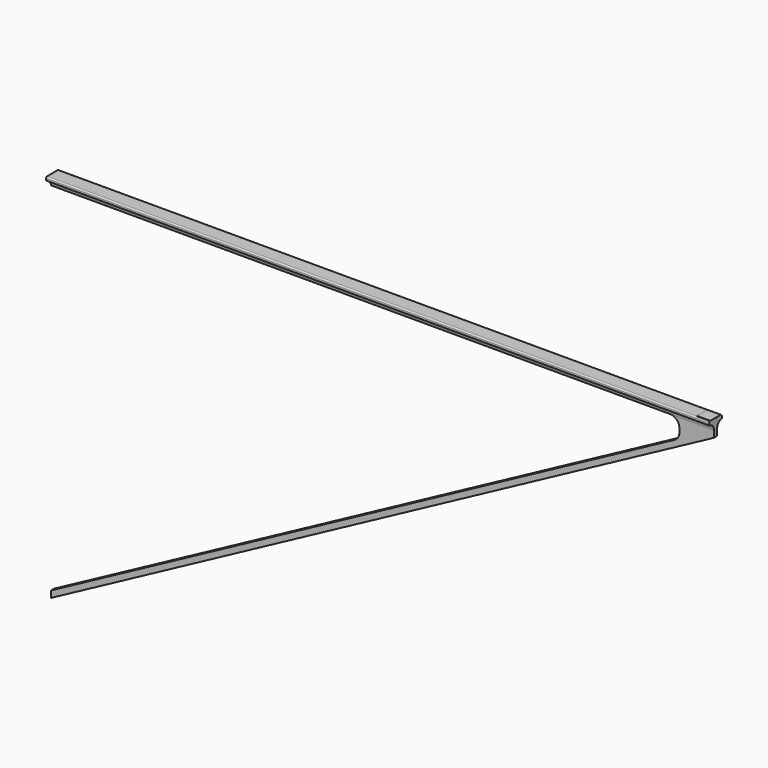
from build123d import *

# Parameters (mm, degrees)
F1_DEPTH      = 502
F3_DEPTH      = 406
F4_DEPTH      = 143
F5_W          = 26.22529459
F5_H          = 3
F6_DEPTH      = 14.25
F6_DEPTH_BACK = 0.8
F8_DEPTH      = 25
F10_DEPTH     = 0.27
F11_R         = 7
F12_R         = 7
F13_T1_DEPTH  = 502
F14_T1_DEPTH  = 502
F15_T1_DEPTH  = 507
F15_T6_DEPTH  = 507
F15_T12_DEPTH = 507
F15_T18_DEPTH = 507
F15_T25_DEPTH = 507
F15_T31_DEPTH = 507


# Not quite as in the source:
# - a fillet or chamfer that OpenCascade refuses, or shapes differently, is made with other operations: its cross-section is extruded or revolved along the edge and cut away or added
# - a feature names something its author has since deleted; it is built from what else it names


with BuildPart() as f1:
    # F0 (on Right) → F1 (new body)
    with BuildSketch(Plane.YZ):
        Polygon((6, 24.6420782059), (-6, 24.6420782059), (-6, 22.1420782059), (-1.5, 22.1420782059), (-1.5, -257.8579217941), (1.5, -257.8579217941), (1.5, 22.1420782059), (6, 22.1420782059), align=None)
    extrude(amount=F1_DEPTH)

    # F2 (on face) → F3 (cut)
    with BuildSketch(Plane.XZ.offset(1.5)):
        Polygon((0, -252.8579217941), (502, 17.1420782059), (0, 17.1420782059), align=None)
    extrude(amount=-F3_DEPTH, mode=Mode.SUBTRACT)

    # F2 (on face) → F4 (cut)
    with BuildSketch(Plane.XZ.offset(1.5)):
        Polygon((502, -257.8579217941), (502, 12.1420782059), (0, -257.8579217941), align=None)
    extrude(amount=-F4_DEPTH, mode=Mode.SUBTRACT)

    # F5 (on face) → F6 (join, two sides)
    with BuildSketch(Plane(origin=(0, 0, 17.1420782059), x_dir=(1, 0, 0), z_dir=(0, 0, -1))) as f6_sk:
        with Locations((488.887352705, 0)):
            Rectangle(F5_W, F5_H)
    extrude(amount=F6_DEPTH)
    extrude(f6_sk.sketch, amount=-F6_DEPTH_BACK)

    # F7 (on face) → F8 (cut)
    with BuildSketch(Plane(origin=(0, 1.5, 0), x_dir=(-1, 0, 0), z_dir=(0, 1, 0))):
        Polygon((-484.8018518519, 2.8920782059), (-502, 12.143202126), (-502, 2.8920782059), align=None)
    extrude(amount=-F8_DEPTH, mode=Mode.SUBTRACT)

    # F9 (on face) → F10 (join)
    with BuildSketch(Plane.XY.offset(24.6420782059)):
        Polygon((501.9800190187, -5.0222751118), (501.9800190187, 4.9777248882), (497.843503952, 4.9777248882), (491.9800190187, 4.9777248882), (491.9800190187, -5.0222751118), (496.5066611767, -5.0222751118), align=None)
    extrude(amount=F10_DEPTH)

    # F11
    f11_edges = [f1.edges().sort_by_distance(p)[0] for p in [
        (475.774705, 0, 17.142078),
    ]]
    fillet(f11_edges, radius=F11_R)

    # F12
    f12_edges = [f1.edges().sort_by_distance(p)[0] for p in [
        (475.774705, 0, 3.03684),
    ]]
    fillet(f12_edges, radius=F12_R)

    # F13: fillet of radius 5 on 1 edges, made by hand

    # F13_s2 → F13_t1 (join)
    with BuildSketch(Plane.YZ):
        with BuildLine():
            ThreePointArc((1.5, 17.1671410204), (2.7919007565, 20.5212429867), (6, 22.1420782059))
            Line((6, 22.1420782059), (1.5, 22.1420782059))
            Line((1.5, 22.1420782059), (1.5, 17.1671410204))
        make_face()
    extrude(amount=F13_T1_DEPTH)

    # F14: fillet of radius 5 on 1 edges, made by hand

    # F14_s2 → F14_t1 (join)
    with BuildSketch(Plane.YZ):
        with BuildLine():
            ThreePointArc((-1.5, 17.1671410204), (-2.7919007565, 20.5212429867), (-6, 22.1420782059))
            Line((-6, 22.1420782059), (-1.5, 22.1420782059))
            Line((-1.5, 22.1420782059), (-1.5, 17.1671410204))
        make_face()
    extrude(amount=F14_T1_DEPTH)

    # F15: fillet of radius 1 on 2 edges, made by hand

    # F15_s2 → F15_t1 (cut)
    with BuildSketch(Plane.YZ.offset(-2.5)):
        with BuildLine():
            ThreePointArc((6, 23.6420782059), (5.7071067812, 24.3491849871), (5, 24.6420782059))
            Line((5, 24.6420782059), (6, 24.6420782059))
            Line((6, 24.6420782059), (6, 23.6420782059))
        make_face()
    extrude(amount=F15_T1_DEPTH, mode=Mode.SUBTRACT)


with BuildPart() as f15_tool4:
    # F15_s5 → F15_t6 (new body)
    with BuildSketch(Plane.YZ.offset(-2.5)):
        with BuildLine():
            ThreePointArc((-5, 24.6420782059), (-5.7071067812, 24.3491849871), (-6, 23.6420782059))
            Line((-6, 23.6420782059), (-6, 24.6420782059))
            Line((-6, 24.6420782059), (-5, 24.6420782059))
        make_face()
    extrude(amount=F15_T6_DEPTH)

    split(bisect_by=Plane.YZ.offset(491.9800190187), keep=Keep.BOTTOM)

    split(bisect_by=Plane.XZ.offset(5.0222751118), keep=Keep.BOTTOM)


with BuildPart() as f1_1:
    add(f1.part)

    # F15_t3: cut F15_tool4
    add(f15_tool4.part, mode=Mode.SUBTRACT)


with BuildPart() as f15_tool10:
    # F15_s11 → F15_t12 (new body)
    with BuildSketch(Plane.YZ.offset(-2.5)):
        with BuildLine():
            ThreePointArc((-5, 24.6420782059), (-5.7071067812, 24.3491849871), (-6, 23.6420782059))
            Line((-6, 23.6420782059), (-6, 24.6420782059))
            Line((-6, 24.6420782059), (-5, 24.6420782059))
        make_face()
    extrude(amount=F15_T12_DEPTH)

    split(bisect_by=Plane.YZ.offset(491.9800190187), keep=Keep.BOTTOM)

    split(bisect_by=Plane.XZ.offset(5.0222751118), keep=Keep.TOP)


with BuildPart() as f1_2:
    add(f1_1.part)

    # F15_t9: cut F15_tool10
    add(f15_tool10.part, mode=Mode.SUBTRACT)


with BuildPart() as f15_tool16:
    # F15_s17 → F15_t18 (new body)
    with BuildSketch(Plane.YZ.offset(-2.5)):
        with BuildLine():
            ThreePointArc((-5, 24.6420782059), (-5.7071067812, 24.3491849871), (-6, 23.6420782059))
            Line((-6, 23.6420782059), (-6, 24.6420782059))
            Line((-6, 24.6420782059), (-5, 24.6420782059))
        make_face()
    extrude(amount=F15_T18_DEPTH)

    split(bisect_by=Plane.YZ.offset(491.9800190187), keep=Keep.TOP)

    split(bisect_by=Plane.YZ.offset(501.9800190187), keep=Keep.BOTTOM)

    split(bisect_by=Plane.XZ.offset(5.0222751118), keep=Keep.TOP)


with BuildPart() as f1_3:
    add(f1_2.part)

    # F15_t15: cut F15_tool16
    add(f15_tool16.part, mode=Mode.SUBTRACT)


with BuildPart() as f15_tool23:
    # F15_s24 → F15_t25 (new body)
    with BuildSketch(Plane.YZ.offset(-2.5)):
        with BuildLine():
            ThreePointArc((-5, 24.6420782059), (-5.7071067812, 24.3491849871), (-6, 23.6420782059))
            Line((-6, 23.6420782059), (-6, 24.6420782059))
            Line((-6, 24.6420782059), (-5, 24.6420782059))
        make_face()
    extrude(amount=F15_T25_DEPTH)

    split(bisect_by=Plane.YZ.offset(501.9800190187), keep=Keep.TOP)

    split(bisect_by=Plane.XZ.offset(5.0222751118), keep=Keep.BOTTOM)


with BuildPart() as f1_4:
    add(f1_3.part)

    # F15_t22: cut F15_tool23
    add(f15_tool23.part, mode=Mode.SUBTRACT)


with BuildPart() as f15_tool29:
    # F15_s30 → F15_t31 (new body)
    with BuildSketch(Plane.YZ.offset(-2.5)):
        with BuildLine():
            ThreePointArc((-5, 24.6420782059), (-5.7071067812, 24.3491849871), (-6, 23.6420782059))
            Line((-6, 23.6420782059), (-6, 24.6420782059))
            Line((-6, 24.6420782059), (-5, 24.6420782059))
        make_face()
    extrude(amount=F15_T31_DEPTH)

    split(bisect_by=Plane.YZ.offset(501.9800190187), keep=Keep.TOP)

    split(bisect_by=Plane.XZ.offset(5.0222751118), keep=Keep.TOP)


with BuildPart() as f1_5:
    add(f1_4.part)

    # F15_t28: cut F15_tool29
    add(f15_tool29.part, mode=Mode.SUBTRACT)


solid = f1_5.part
